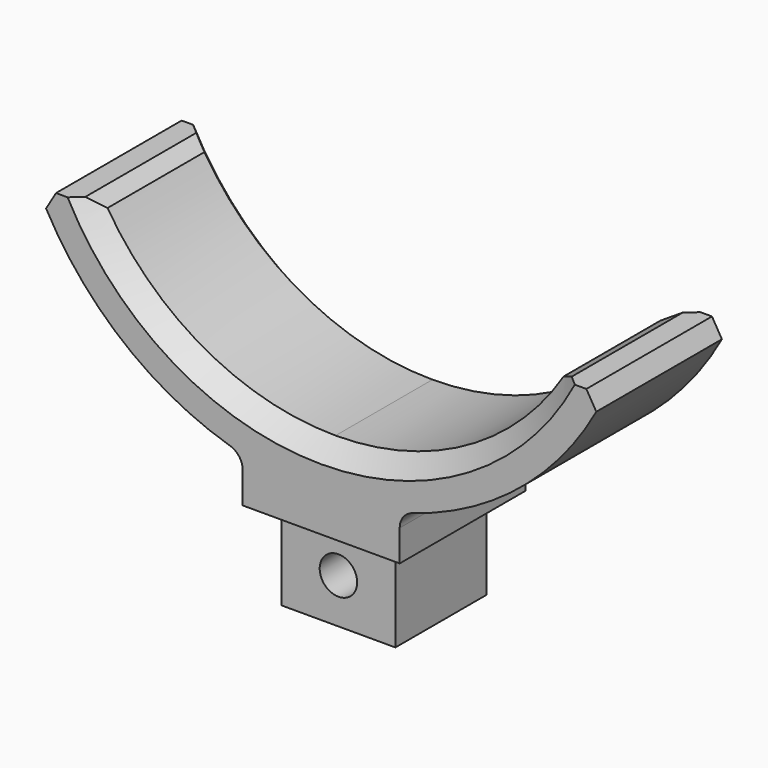
from build123d import *

# Parameters (mm, degrees)
F0_W        = 16.129
F0_H        = 25.4
F1_DEPTH    = 44.45
F2_W        = 32.258
F2_H        = 6.096
F3_DEPTH    = 25.4
F4_R        = 5.30225
F5_DEPTH    = 38.355
F6_R        = 5.08
F7_T1_DEPTH = 59.6994752683
F7_T4_ANGLE = 139.6602442287
F7_T6_ANGLE = 139.6602442287
F8_T1_DEPTH = 71.752763855


# Not quite as in the source:
# - a fillet or chamfer that OpenCascade refuses, or shapes differently, is made with other operations: its cross-section is extruded or revolved along the edge and cut away or added


with BuildPart() as f1:
    # F0 (on Front) → F1 (new body)
    with BuildSketch(Plane.XZ):
        with BuildLine():
            ThreePointArc((0, -76.2), (-38.1, -65.9911357684), (-65.9911357684, -38.1))
            Line((-65.9911357684, -38.1), (-80.3218525683, -38.1))
            ThreePointArc((-80.3218525683, -38.1), (-56.6075409411, -68.5477666201), (-22.225, -86.0770548695))
            Line((-22.225, -86.0770548695), (0, -86.0770548695))
            Line((0, -86.0770548695), (0, -76.2))
        make_face()
        with BuildLine():
            Line((80.3218525683, -38.1), (65.9911357684, -38.1))
            ThreePointArc((65.9911357684, -38.1), (38.1, -65.9911357684), (0, -76.2))
            Line((0, -76.2), (0, -86.0770548695))
            Line((0, -86.0770548695), (22.225, -86.0770548695))
            ThreePointArc((22.225, -86.0770548695), (56.6075409411, -68.5477666201), (80.3218525683, -38.1))
        make_face()
        with BuildLine():
            Line((22.225, -98.7770548695), (22.225, -86.0770548695))
            ThreePointArc((22.225, -86.0770548695), (11.2017816017, -88.1914399982), (0, -88.9))
            Line((0, -88.9), (0, -98.7770548695))
            Line((0, -98.7770548695), (16.129, -98.7770548695))
            Line((16.129, -98.7770548695), (22.225, -98.7770548695))
        make_face()
        with BuildLine():
            ThreePointArc((0, -88.9), (-11.2017816017, -88.1914399982), (-22.225, -86.0770548695))
            Line((-22.225, -86.0770548695), (-22.225, -98.7770548695))
            Line((-22.225, -98.7770548695), (-16.129, -98.7770548695))
            Line((-16.129, -98.7770548695), (0, -98.7770548695))
            Line((0, -98.7770548695), (0, -88.9))
        make_face()
        with Locations((8.0645, -111.4770548695)):
            Rectangle(F0_W, F0_H)
        with Locations((-8.0645, -111.4770548695)):
            Rectangle(F0_W, F0_H)
        with BuildLine():
            Line((22.225, -86.0770548695), (0, -86.0770548695))
            Line((0, -86.0770548695), (0, -88.9))
            ThreePointArc((0, -88.9), (11.2017816017, -88.1914399982), (22.225, -86.0770548695))
        make_face()
        with BuildLine():
            Line((0, -88.9), (0, -86.0770548695))
            Line((0, -86.0770548695), (-22.225, -86.0770548695))
            ThreePointArc((-22.225, -86.0770548695), (-11.2017816017, -88.1914399982), (0, -88.9))
        make_face()
    extrude(amount=F1_DEPTH)

    # F2 (on face) → F3 (cut)
    with BuildSketch(Plane(origin=(0, 0, -124.1770548695), x_dir=(1, 0, 0), z_dir=(0, 0, -1))):
        with Locations((0, 41.402)):
            Rectangle(F2_W, F2_H)
        with Locations((0, 3.048)):
            Rectangle(F2_W, F2_H)
    extrude(amount=-F3_DEPTH, mode=Mode.SUBTRACT)

    # F4 (on face) → F5 (cut, through all)
    with BuildSketch(Plane.XZ.offset(38.354)):
        with Locations((0, -111.4770548695)):
            Circle(F4_R)
    extrude(amount=-F5_DEPTH, mode=Mode.SUBTRACT)

    # F6
    f6_edges = [f1.edges().sort_by_distance(p)[0] for p in [
        (-22.225, -22.225, -86.077055),
        (22.225, -22.225, -86.077055),
    ]]
    fillet(f6_edges, radius=F6_R)

    # F7: chamfer of 5.08 on 4 edges, made by hand

    # F7_s2 → F7_t1 (cut)
    with BuildSketch(Plane.XZ.offset(-7.6247376341)):
        with BuildLine():
            Line((-68.8616438956, -38.1), (-64.5577911521, -40.48125))
            ThreePointArc((-64.5577911521, -40.48125), (-65.2398633811, -39.3725821609), (-65.9911357684, -38.1))
            Line((-65.9911357684, -38.1), (-68.8616438956, -38.1))
        make_face()
        with BuildLine():
            Line((64.5577911521, -40.48125), (68.8616438956, -38.1))
            Line((68.8616438956, -38.1), (65.9911357684, -38.1))
            ThreePointArc((65.9911357684, -38.1), (65.2398633811, -39.3725821609), (64.5577911521, -40.48125))
        make_face()
    extrude(amount=F7_T1_DEPTH, mode=Mode.SUBTRACT)

    # F7_s3 → F7_t4 (revolve, cut)
    with BuildSketch(Plane(origin=(0, 0, 0), x_dir=(0, 1, 0), z_dir=(0.3448047573, 0, 0.9386744267))):
        Polygon((-44.45, -81.28), (-39.37, -76.2), (-44.45, -76.2), align=None)
    revolve(axis=Axis((0, -44.45, 0), (0, 1, 0)), revolution_arc=F7_T4_ANGLE, mode=Mode.SUBTRACT)

    # F7_s5 → F7_t6 (revolve, cut)
    with BuildSketch(Plane(origin=(0, 0, 0), x_dir=(0, 1, 0), z_dir=(0.3448047573, 0, 0.9386744267))):
        Polygon((0, -81.28), (-5.08, -76.2), (0, -76.2), align=None)
    revolve(axis=Axis((0, 0, 0), (0, 1, 0)), revolution_arc=F7_T6_ANGLE, mode=Mode.SUBTRACT)

    # F8: chamfer of 5.08 on 2 edges, made by hand

    # F8_s2 → F8_t1 (cut)
    with BuildSketch(Plane.XZ.offset(-13.6513819275)):
        with BuildLine():
            Line((74.966768006, -37.9250746392), (77.988352908, -43.0368427057))
            Line((77.988352908, -43.0368427057), (78.0773642839, -43.0858277541))
            ThreePointArc((78.0773642839, -43.0858277541), (79.2049019091, -40.5939443284), (80.4136489712, -38.1435428571))
            Line((80.4136489712, -38.1435428571), (80.3218525683, -37.9984))
            ThreePointArc((80.3218525683, -37.9984), (77.6443102871, -37.9984), (74.966768006, -37.8234746392))
            Line((74.966768006, -37.8234746392), (74.966768006, -37.9250746392))
        make_face()
        with BuildLine():
            Line((-77.988352908, -43.0368427057), (-74.966768006, -37.9250746392))
            Line((-74.966768006, -37.9250746392), (-74.966768006, -37.8234746392))
            ThreePointArc((-74.966768006, -37.8234746392), (-77.6443102871, -37.9984), (-80.3218525683, -37.9984))
            Line((-80.3218525683, -37.9984), (-80.4136489712, -38.1435428571))
            ThreePointArc((-80.4136489712, -38.1435428571), (-79.2049019091, -40.5939443284), (-78.0773642839, -43.0858277541))
            Line((-78.0773642839, -43.0858277541), (-77.988352908, -43.0368427057))
        make_face()
    extrude(amount=F8_T1_DEPTH, mode=Mode.SUBTRACT)


solid = f1.part
